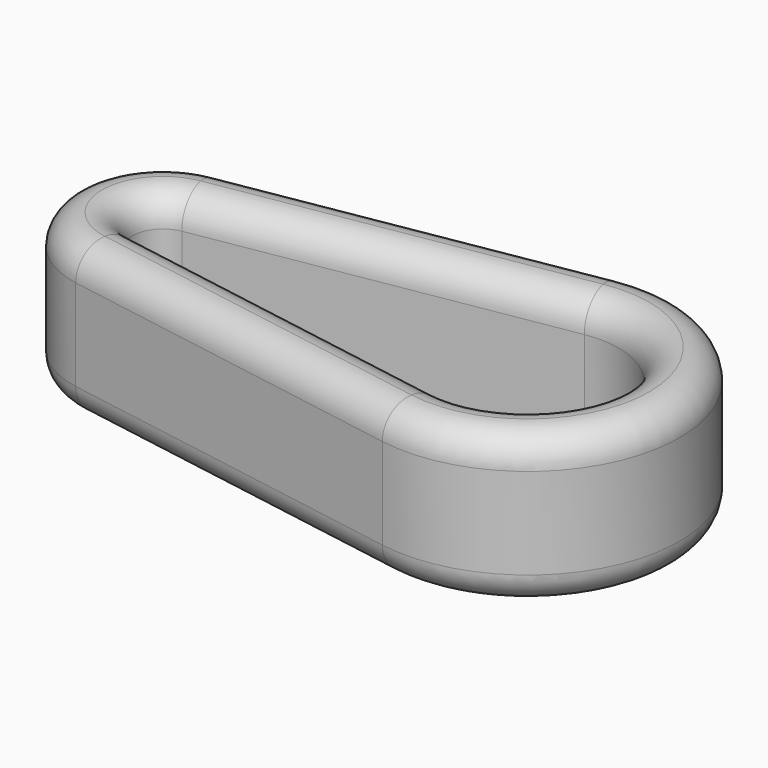
from build123d import *

# Parameters (mm, degrees)
F1_DEPTH = 25
F2_R     = 5
F3_R     = 4.99999
F4_R     = 4.99999


# Not quite as in the source:
# - a fillet or chamfer is up to 0.001 mm smaller than in the source, because OpenCascade refuses the exact size


with BuildPart() as f1:
    # F0 (on Top) → F1 (new body)
    with BuildSketch(Plane.XY):
        with BuildLine():
            Line((-4.1666666667, 24.6503324296), (-62.5, 14.7901994577))
            ThreePointArc((-62.5, 14.7901994577), (-75, 0), (-62.5, -14.7901994577))
            Line((-62.5, -14.7901994577), (-4.1666666667, -24.6503324296))
            ThreePointArc((-4.1666666667, -24.6503324296), (25, 0), (-4.1666666667, 24.6503324296))
        make_face()
        with BuildLine():
            Line((-60.8333333333, 4.9300664859), (-2.5, 14.7901994577))
            ThreePointArc((-2.5, 14.7901994577), (15, 0), (-2.5, -14.7901994577))
            Line((-2.5, -14.7901994577), (-60.8333333333, -4.9300664859))
            ThreePointArc((-60.8333333333, -4.9300664859), (-65, 0), (-60.8333333333, 4.9300664859))
        make_face(mode=Mode.SUBTRACT)
    extrude(amount=F1_DEPTH)

    # F2
    f2_edges = [f1.edges().sort_by_distance(p)[0] for p in [
        (-33.333333, -19.720266, 25),
        (25, 0, 25),
        (-33.333333, -19.720266, 0),
        (25, 0, 0),
    ]]
    fillet(f2_edges, radius=F2_R)

    # F3 (radius 5 in the source; OpenCascade refuses exactly that, so slightly less here)
    f3_edges = [f1.edges().sort_by_distance(p)[0] for p in [
        (-31.666667, 9.860133, 25),
    ]]
    fillet(f3_edges, radius=F3_R)

    # F4 (radius 5 in the source; OpenCascade refuses exactly that, so slightly less here)
    f4_edges = [f1.edges().sort_by_distance(p)[0] for p in [
        (15, 0, 0),
        (-31.666667, 9.860133, 0),
    ]]
    fillet(f4_edges, radius=F4_R)


solid = f1.part
